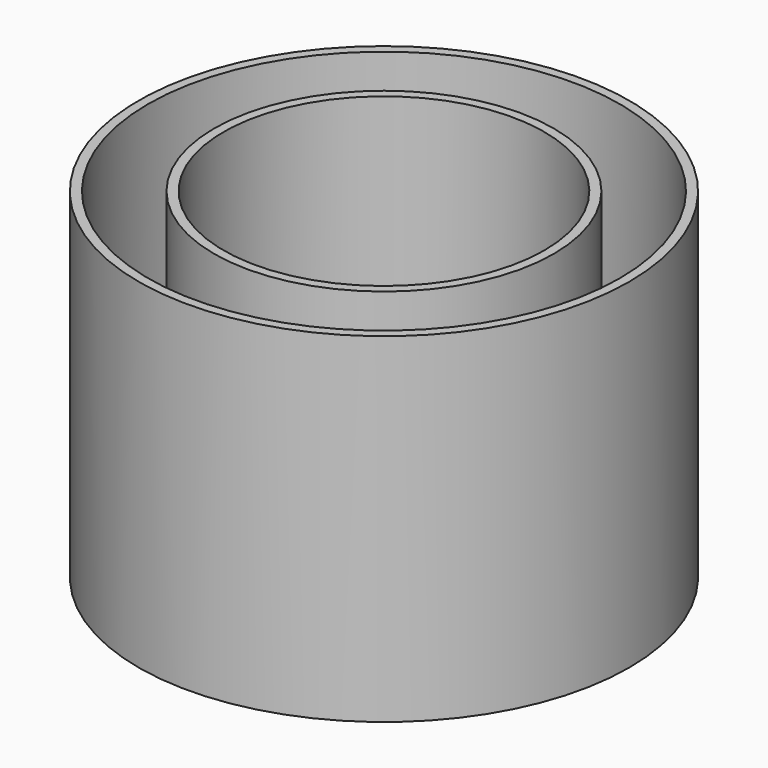
from build123d import *

# Parameters (mm, degrees)
F0_R     = 65
F0_R_2   = 62.5
F1_DEPTH = 90
F0_R_3   = 45
F0_R_4   = 42.5
F2_W     = 130
F2_H     = 65
F3_DEPTH = 250


# Not quite as in the source:
# - an extrude ends at something that could not be found from the text; its depth is read off the source's solid


with BuildPart() as f1:
    # F0 (on Top) → F1 (new body)
    with BuildSketch(Plane.XY):
        Circle(F0_R)
        Circle(F0_R_2, mode=Mode.SUBTRACT)
    extrude(amount=F1_DEPTH)

    # F2 (on Top) → F3 (cut, through all)
    with BuildSketch(Plane.XY):
        with Locations((0, -32.5)):
            Rectangle(F2_W, F2_H)
    extrude(amount=-F3_DEPTH, mode=Mode.SUBTRACT)


with BuildPart() as f1b:
    # F0 (on Top) → F1, piece 2 (new body)
    with BuildSketch(Plane.XY):
        Circle(F0_R_3)
        Circle(F0_R_4, mode=Mode.SUBTRACT)
    extrude(amount=F1_DEPTH)


solid = Compound([f1.part, f1b.part])
